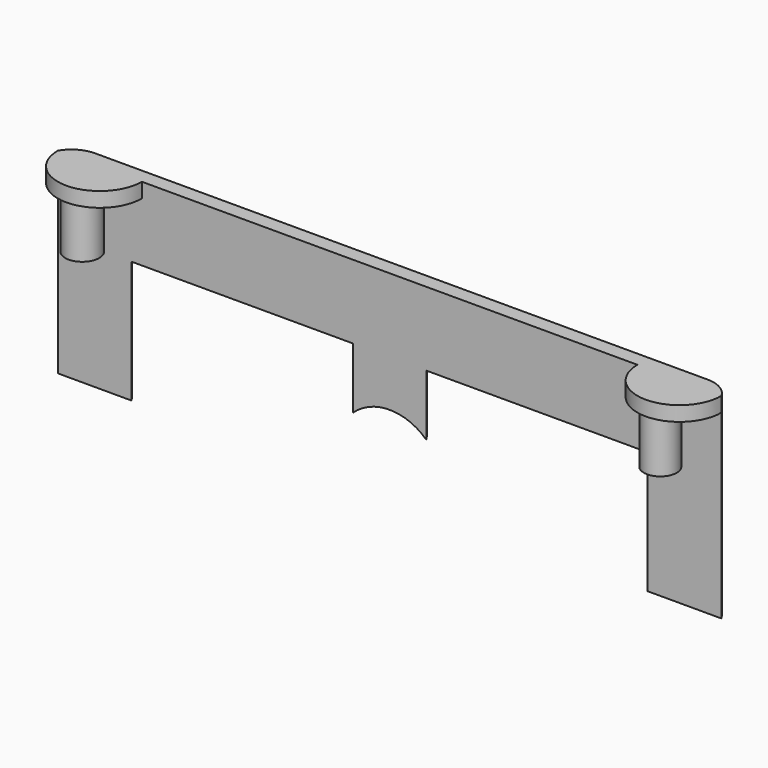
from build123d import *

# Parameters (mm, degrees)
F1_DEPTH     = 2.54
F3_DEPTH     = 2.54
F4_R         = 2.9314454593
F5_R         = 2.8319389427
F6_DEPTH     = 8.89
F8_DEPTH     = 25.4
F9_T1_DEPTH  = 38.1
F9_T3_DEPTH  = 38.1
F9_T5_DEPTH  = 21.5282681004
F9_T7_DEPTH  = 32.0580135728
F9_T9_DEPTH  = 55.7565362009
F9_T11_DEPTH = 34.6970452561
F9_T13_DEPTH = 34.6970452561
F9_T16_ANGLE = 223.4050528115
F9_T21_DEPTH = 49.0985226281
F9_T25_DEPTH = 32.5267907285
F9_T32_DEPTH = 32.0580135728
F9_T37_DEPTH = 49.0985226281
F9_T44_DEPTH = 49.0985226281
F9_T48_DEPTH = 32.0580135728
F9_T56_DEPTH = 32.5267907285
F9_T60_DEPTH = 49.0985226281
F10_R        = 1.4567648878
F10_R_2      = 1.5876943873
F11_DEPTH    = 0.508
F12_R        = 0.6244535606
F12_R_2      = 0.645662674
F13_DEPTH    = 0.254


# Not quite as in the source:
# - a fillet or chamfer that OpenCascade refuses, or shapes differently, is made with other operations: its cross-section is extruded or revolved along the edge and cut away or added


with BuildPart() as f1:
    # F0 (on Front) → F1 (new body)
    with BuildSketch(Plane.XZ):
        Polygon((27.5468391635, 41.7749450469), (-86.7531608365, 41.7749450469), (-86.7531608365, 8.0154541022), (-74.0531608365, 8.0154541022), (-74.0531608365, 29.0749450469), (-35.9531608365, 29.0749450469), (-35.9531608365, 8.0154541022), (-23.2531608365, 8.0154541022), (-23.2531608365, 29.0749450469), (14.8468391635, 29.0749450469), (14.8468391635, 8.0154541022), (27.5468391635, 8.0154541022), align=None)
    extrude(amount=F1_DEPTH)

    # F2 (on face) → F3 (join)
    with BuildSketch(Plane.XY.offset(41.7749450469)):
        with BuildLine():
            Line((27.5468391635, -2.54), (13.0688391635, -2.54))
            ThreePointArc((13.0688391635, -2.54), (20.3078391635, -9.779), (27.5468391635, -2.54))
        make_face()
        with BuildLine():
            Line((-72.2751608365, -2.54), (-86.7531608365, -2.54))
            ThreePointArc((-86.7531608365, -2.54), (-79.5141608365, -9.779), (-72.2751608365, -2.54))
        make_face()
    extrude(amount=-F3_DEPTH)

    # F4 (on face) + F5 (on face) → F6 (join)
    with BuildSketch(Plane(origin=(0, 0, 39.2349450469), x_dir=(1, 0, 0), z_dir=(0, 0, -1))):
        with Locations((-79.5141608365, 6.3278437592)):
            Circle(F4_R)
    with BuildSketch(Plane(origin=(0, 0, 39.2349450469), x_dir=(1, 0, 0), z_dir=(0, 0, -1))):
        with Locations((20.3078391635, 6.6598863341)):
            Circle(F5_R)
    extrude(amount=F6_DEPTH)

    # F7 (on face) → F8 (cut)
    with BuildSketch(Plane.XZ.offset(2.54)):
        with BuildLine():
            Line((-23.2531608365, 8.0154541022), (-23.2531608365, 18.5451995745))
            ThreePointArc((-23.2531608365, 18.5451995745), (-29.6031608365, 21.0747577819), (-35.9531608365, 18.5451995745))
            Line((-35.9531608365, 18.5451995745), (-35.9531608365, 8.0154541022))
            Line((-35.9531608365, 8.0154541022), (-23.2531608365, 8.0154541022))
        make_face()
    extrude(amount=-F8_DEPTH, mode=Mode.SUBTRACT)

    # F9: fillet of radius 5.08 on 11 edges, made by hand

    # F9_s2 → F9_t1 (cut)
    with BuildSketch(Plane.YZ.offset(-23.2531608365)):
        with BuildLine():
            ThreePointArc((0, 33.4743540981), (-0.6805909488, 30.9343540981), (-2.54, 29.0749450469))
            Line((-2.54, 29.0749450469), (0, 29.0749450469))
            Line((0, 29.0749450469), (0, 33.4743540981))
        make_face()
    extrude(amount=F9_T1_DEPTH, mode=Mode.SUBTRACT)

    # F9_s4 → F9_t3 (cut)
    with BuildSketch(Plane.YZ.offset(-74.0531608365)):
        with BuildLine():
            ThreePointArc((0, 33.4743540981), (-0.6805909488, 30.9343540981), (-2.54, 29.0749450469))
            Line((-2.54, 29.0749450469), (0, 29.0749450469))
            Line((0, 29.0749450469), (0, 33.4743540981))
        make_face()
    extrude(amount=F9_T3_DEPTH, mode=Mode.SUBTRACT)

    # F9_s6 → F9_t5 (cut)
    with BuildSketch(Plane.XY.offset(7.5466769465)):
        with BuildLine():
            ThreePointArc((-31.5537517853, 0), (-34.0937517853, -0.6805909488), (-35.9531608365, -2.54))
            Line((-35.9531608365, -2.54), (-35.9531608365, 0))
            Line((-35.9531608365, 0), (-31.5537517853, 0))
        make_face()
        with BuildLine():
            ThreePointArc((-27.6525698878, 0), (-25.1125698878, -0.6805909488), (-23.2531608365, -2.54))
            Line((-23.2531608365, -2.54), (-23.2531608365, 0))
            Line((-23.2531608365, 0), (-27.6525698878, 0))
        make_face()
    extrude(amount=F9_T5_DEPTH, mode=Mode.SUBTRACT)

    # F9_s8 → F9_t7 (cut)
    with BuildSketch(Plane.XY.offset(-2.9830685259)):
        with BuildLine():
            ThreePointArc((19.2462482147, 0), (16.7062482147, -0.6805909488), (14.8468391635, -2.54))
            Line((14.8468391635, -2.54), (14.8468391635, 0))
            Line((14.8468391635, 0), (19.2462482147, 0))
        make_face()
        with BuildLine():
            ThreePointArc((-78.4525698878, 0), (-75.9125698878, -0.6805909488), (-74.0531608365, -2.54))
            Line((-74.0531608365, -2.54), (-74.0531608365, 0))
            Line((-74.0531608365, 0), (-78.4525698878, 0))
        make_face()
    extrude(amount=F9_T7_DEPTH, mode=Mode.SUBTRACT)

    # F9_s10 → F9_t9 (cut)
    with BuildSketch(Plane.XY.offset(-2.9830685259)):
        with BuildLine():
            ThreePointArc((27.5468391635, -2.54), (25.6874301122, -0.6805909488), (23.1474301122, 0))
            Line((23.1474301122, 0), (27.5468391635, 0))
            Line((27.5468391635, 0), (27.5468391635, -2.54))
        make_face()
        with BuildLine():
            ThreePointArc((-86.7531608365, -2.54), (-84.8937517853, -0.6805909488), (-82.3537517853, 0))
            Line((-82.3537517853, 0), (-86.7531608365, 0))
            Line((-86.7531608365, 0), (-86.7531608365, -2.54))
        make_face()
    extrude(amount=F9_T9_DEPTH, mode=Mode.SUBTRACT)

    # F9_s12 → F9_t11 (cut)
    with BuildSketch(Plane.YZ.offset(-97.7516834646)):
        with BuildLine():
            ThreePointArc((0, 12.4148631534), (-0.6805909488, 9.8748631534), (-2.54, 8.0154541022))
            Line((-2.54, 8.0154541022), (0, 8.0154541022))
            Line((0, 8.0154541022), (0, 12.4148631534))
        make_face()
    extrude(amount=F9_T11_DEPTH, mode=Mode.SUBTRACT)

    # F9_s14 → F9_t13 (cut)
    with BuildSketch(Plane.YZ.offset(3.8483165354)):
        with BuildLine():
            ThreePointArc((0, 12.4148631534), (-0.6805909488, 9.8748631534), (-2.54, 8.0154541022))
            Line((-2.54, 8.0154541022), (0, 8.0154541022))
            Line((0, 8.0154541022), (0, 12.4148631534))
        make_face()
    extrude(amount=F9_T13_DEPTH, mode=Mode.SUBTRACT)

    # F9_s15 → F9_t16 (revolve, cut)
    with BuildSketch(Plane(origin=(0.0198149882, 0, 0.0497864763), x_dir=(0, 1, 0), z_dir=(-0.3697877262, 0, -0.929116267))):
        with BuildLine():
            ThreePointArc((0, -18.2485055237), (-0.6805909488, -20.7885055237), (-2.54, -22.6479145749))
            Line((-2.54, -22.6479145749), (0, -22.6479145749))
            Line((0, -22.6479145749), (0, -18.2485055237))
        make_face()
    revolve(axis=Axis((-29.6031608365, 0, 11.8397133801), (0, -1, 0)), revolution_arc=F9_T16_ANGLE, mode=Mode.SUBTRACT)


with BuildPart() as f9_tool19:
    # F9_s20 → F9_t21 (new body)
    with BuildSketch(Plane.YZ.offset(-34.2516834646)):
        with BuildLine():
            ThreePointArc((0, 33.4743540981), (-0.6805909488, 30.9343540981), (-2.54, 29.0749450469))
            Line((-2.54, 29.0749450469), (0, 29.0749450469))
            Line((0, 29.0749450469), (0, 33.4743540981))
        make_face()
    extrude(amount=F9_T21_DEPTH)

    split(bisect_by=Plane.YZ.offset(-23.2531608365), keep=Keep.BOTTOM)


with BuildPart() as f9_tool23:
    # F9_s24 → F9_t25 (new body)
    with BuildSketch(Plane.XY.offset(7.5466769465)):
        with BuildLine():
            ThreePointArc((-27.6525698878, 0), (-25.1125698878, -0.6805909488), (-23.2531608365, -2.54))
            Line((-23.2531608365, -2.54), (-23.2531608365, 0))
            Line((-23.2531608365, 0), (-27.6525698878, 0))
        make_face()
    extrude(amount=F9_T25_DEPTH)

    split(bisect_by=Plane.XY.offset(29.0749450469), keep=Keep.TOP)


with BuildPart() as f9_tool19_1:
    add(f9_tool19.part)

    # F9_t27: intersect F9_tool23
    add(f9_tool23.part, mode=Mode.INTERSECT)


with BuildPart() as f1_1:
    add(f1.part)

    # F9_t17: cut F9_tool19
    add(f9_tool19_1.part, mode=Mode.SUBTRACT)


with BuildPart() as f9_tool30:
    # F9_s31 → F9_t32 (new body)
    with BuildSketch(Plane.XY.offset(40.073467675)):
        with BuildLine():
            ThreePointArc((19.2462482147, 0), (16.7062482147, -0.6805909488), (14.8468391635, -2.54))
            Line((14.8468391635, -2.54), (14.8468391635, 0))
            Line((14.8468391635, 0), (19.2462482147, 0))
        make_face()
    extrude(amount=-F9_T32_DEPTH)

    split(bisect_by=Plane.XY.offset(39.2349450469), keep=Keep.BOTTOM)

    split(bisect_by=Plane.XY.offset(29.0749450469), keep=Keep.TOP)


with BuildPart() as f9_tool35:
    # F9_s36 → F9_t37 (new body)
    with BuildSketch(Plane.YZ.offset(-23.2531608365)):
        with BuildLine():
            ThreePointArc((0, 33.4743540981), (-0.6805909488, 30.9343540981), (-2.54, 29.0749450469))
            Line((-2.54, 29.0749450469), (0, 29.0749450469))
            Line((0, 29.0749450469), (0, 33.4743540981))
        make_face()
    extrude(amount=F9_T37_DEPTH)

    split(bisect_by=Plane.YZ.offset(14.8468391635), keep=Keep.TOP)


with BuildPart() as f9_tool30_1:
    add(f9_tool30.part)

    # F9_t39: intersect F9_tool35
    add(f9_tool35.part, mode=Mode.INTERSECT)


with BuildPart() as f1_2:
    add(f1_1.part)

    # F9_t28: cut F9_tool30
    add(f9_tool30_1.part, mode=Mode.SUBTRACT)


with BuildPart() as f9_tool42:
    # F9_s43 → F9_t44 (new body)
    with BuildSketch(Plane.YZ.offset(-85.0516834646)):
        with BuildLine():
            ThreePointArc((0, 33.4743540981), (-0.6805909488, 30.9343540981), (-2.54, 29.0749450469))
            Line((-2.54, 29.0749450469), (0, 29.0749450469))
            Line((0, 29.0749450469), (0, 33.4743540981))
        make_face()
    extrude(amount=F9_T44_DEPTH)

    split(bisect_by=Plane.YZ.offset(-74.0531608365), keep=Keep.BOTTOM)


with BuildPart() as f9_tool46:
    # F9_s47 → F9_t48 (new body)
    with BuildSketch(Plane.XY.offset(8.0154541022)):
        with BuildLine():
            ThreePointArc((-78.4525698878, 0), (-75.9125698878, -0.6805909488), (-74.0531608365, -2.54))
            Line((-74.0531608365, -2.54), (-74.0531608365, 0))
            Line((-74.0531608365, 0), (-78.4525698878, 0))
        make_face()
    extrude(amount=F9_T48_DEPTH)

    split(bisect_by=Plane.XY.offset(29.0749450469), keep=Keep.TOP)

    split(bisect_by=Plane.XY.offset(39.2349450469), keep=Keep.BOTTOM)


with BuildPart() as f9_tool42_1:
    add(f9_tool42.part)

    # F9_t51: intersect F9_tool46
    add(f9_tool46.part, mode=Mode.INTERSECT)


with BuildPart() as f1_3:
    add(f1_2.part)

    # F9_t40: cut F9_tool42
    add(f9_tool42_1.part, mode=Mode.SUBTRACT)


with BuildPart() as f9_tool54:
    # F9_s55 → F9_t56 (new body)
    with BuildSketch(Plane.XY.offset(40.073467675)):
        with BuildLine():
            ThreePointArc((-31.5537517853, 0), (-34.0937517853, -0.6805909488), (-35.9531608365, -2.54))
            Line((-35.9531608365, -2.54), (-35.9531608365, 0))
            Line((-35.9531608365, 0), (-31.5537517853, 0))
        make_face()
    extrude(amount=-F9_T56_DEPTH)

    split(bisect_by=Plane.XY.offset(29.0749450469), keep=Keep.TOP)


with BuildPart() as f9_tool58:
    # F9_s59 → F9_t60 (new body)
    with BuildSketch(Plane.YZ.offset(-74.0531608365)):
        with BuildLine():
            ThreePointArc((0, 33.4743540981), (-0.6805909488, 30.9343540981), (-2.54, 29.0749450469))
            Line((-2.54, 29.0749450469), (0, 29.0749450469))
            Line((0, 29.0749450469), (0, 33.4743540981))
        make_face()
    extrude(amount=F9_T60_DEPTH)

    split(bisect_by=Plane.YZ.offset(-35.9531608365), keep=Keep.TOP)


with BuildPart() as f9_tool54_1:
    add(f9_tool54.part)

    # F9_t62: intersect F9_tool58
    add(f9_tool58.part, mode=Mode.INTERSECT)


with BuildPart() as f1_4:
    add(f1_3.part)

    # F9_t52: cut F9_tool54
    add(f9_tool54_1.part, mode=Mode.SUBTRACT)

    # F10 (on Front) → F11 (cut)
    with BuildSketch(Plane.XZ):
        with Locations((21.32573165, 15.5286919326)):
            Circle(F10_R)
        with Locations((-80.219194293, 15.5286919326)):
            Circle(F10_R_2)
    extrude(amount=F11_DEPTH, mode=Mode.SUBTRACT)

    # F12 (on face) → F13 (join)
    with BuildSketch(Plane(origin=(0, -0.508, 0), x_dir=(-1, 0, 0), z_dir=(0, 1, 0))):
        with Locations((-21.32573165, 15.5286919326)):
            Circle(F12_R)
        with Locations((80.0827890635, 15.5286919326)):
            Circle(F12_R_2)
    extrude(amount=F13_DEPTH)


solid = f1_4.part
